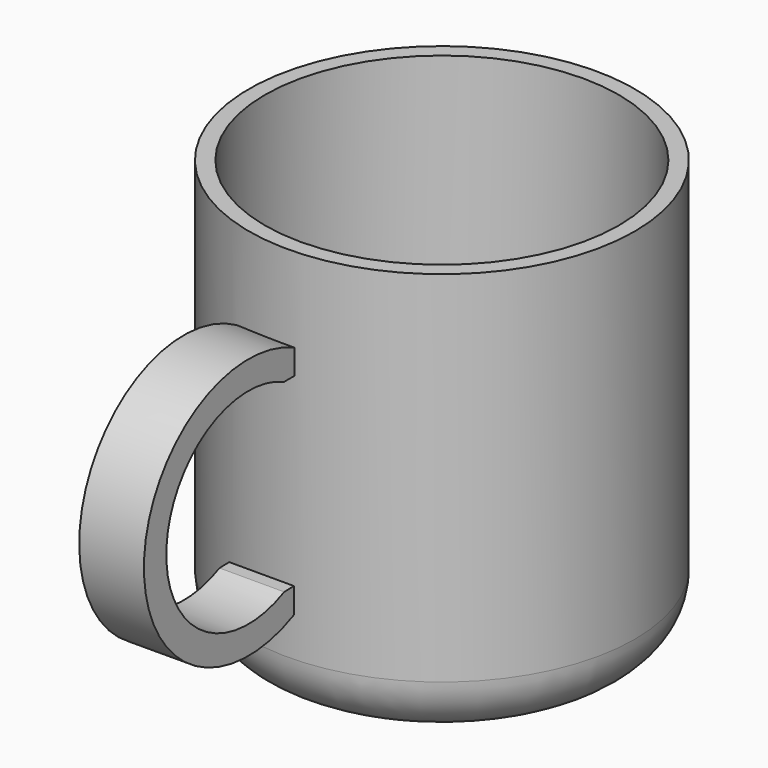
from build123d import *

# Parameters (mm, degrees)
F0_R     = 48.2949752594
F1_DEPTH = 104.394
F2_R     = 14.4852813742
F3_T     = -4
F6_DEPTH = 8.1


# Not quite as in the source:
# - a feature of the source that left no trace in its solid (it failed there, or was rolled back) is left out


with BuildPart() as f1:
    # F0 (on Top) → F1 (new body)
    with BuildSketch(Plane.XY):
        with Locations((6.398510754, 6.8632753311)):
            Circle(F0_R)
    extrude(amount=F1_DEPTH)

    # F2
    f2_edges = [f1.edges().sort_by_distance(p)[0] for p in [
        (-41.896465, 6.863275, 0),
    ]]
    fillet(f2_edges, radius=F2_R)

    # F3
    f3_openings = [f1.faces().sort_by_distance(p)[0] for p in [
        (6.398511, 6.863275, 104.394),
    ]]
    offset(amount=F3_T, openings=f3_openings)

    # F5 (on Right) → F6 (join, symmetric)
    with BuildSketch(Plane.YZ):
        with BuildLine():
            Line((-38.8429239392, 77.0174632754), (-38.8429239392, 81.8370801914))
            ThreePointArc((-38.8429239392, 81.8370801914), (-88.478602233, 55.4130888204), (-41.5783710778, 24.392189458))
            Line((-41.5783710778, 24.392189458), (-41.5783710778, 30.7706389778))
            Line((-41.5783710778, 30.7706389778), (-44.6209337434, 30.6963794891))
            ThreePointArc((-44.6209337434, 30.6963794891), (-81.5156325698, 53.8569213822), (-44.6209337434, 77.0174632754))
            Line((-44.6209337434, 77.0174632754), (-38.8429239392, 77.0174632754))
        make_face()
    extrude(amount=F6_DEPTH, both=True)


solid = f1.part
